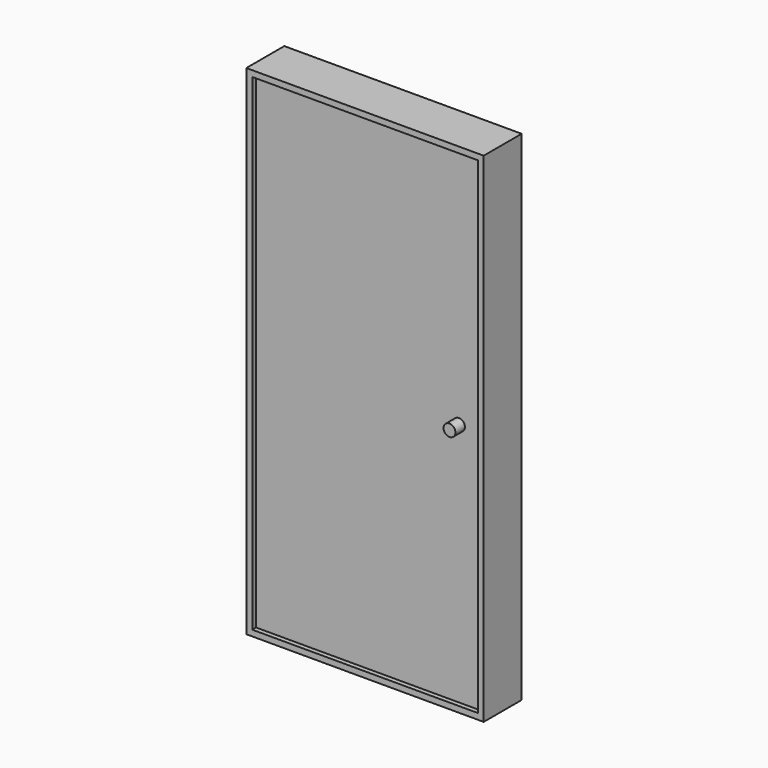
from build123d import *

# Parameters (mm, degrees)
F0_W          = 95
F0_H          = 205
F1_DEPTH      = 10
F1_DEPTH_BACK = 10
F2_DEPTH      = 8
F2_DEPTH_BACK = 8
F3_R          = 2.5
F4_DEPTH      = 5


with BuildPart() as f1:
    # F0 (on Front) → F1 (new body, two sides)
    with BuildSketch(Plane.XZ) as f1_sk:
        Polygon((-97.5, 185), (-100, 185), (-100, 182.5), (-100, -25), (-2.5, -25), (0, -25), (0, -22.5), (0, 185), align=None)
        with Locations((-50, 80)):
            Rectangle(F0_W, F0_H, mode=Mode.SUBTRACT)
    extrude(amount=F1_DEPTH)
    extrude(f1_sk.sketch, amount=-F1_DEPTH_BACK)

    # F0 (on Front) → F2 (join, two sides)
    with BuildSketch(Plane.XZ) as f2_sk:
        with Locations((-50, 80)):
            Rectangle(F0_W, F0_H)
    extrude(amount=F2_DEPTH)
    extrude(f2_sk.sketch, amount=-F2_DEPTH_BACK)


with BuildPart() as f4:
    # F3 (on face) → F4 (new body)
    with BuildSketch(Plane.XZ.offset(8)):
        with Locations((-12.0185082778, 80.4874971509)):
            Circle(F3_R)
    extrude(amount=F4_DEPTH)


solid = Compound([f1.part, f4.part])
